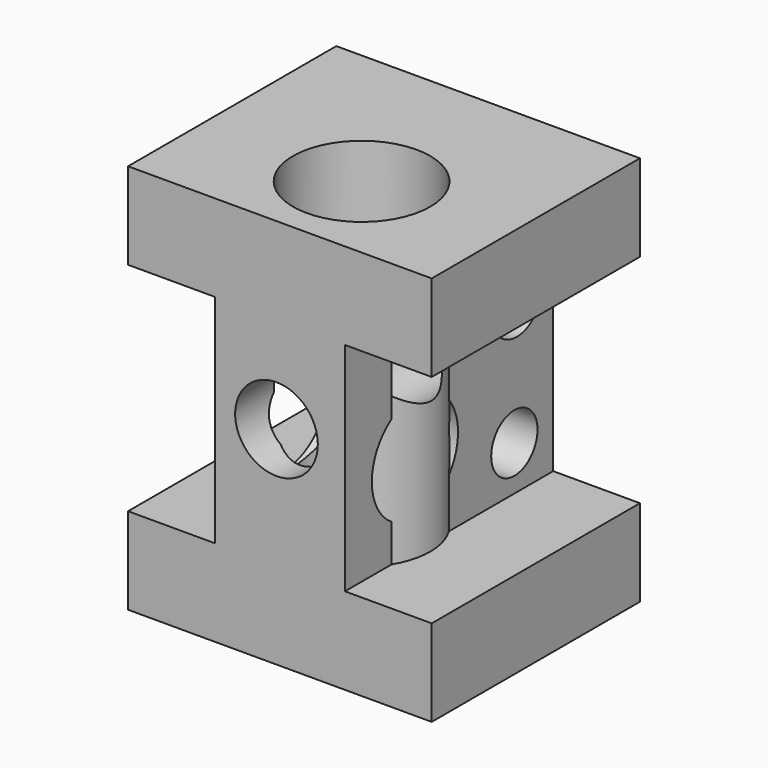
from build123d import *

# Parameters (mm, degrees)
F1_DEPTH  = 76.2
F2_R      = 15.7651741011
F3_DEPTH  = 63.501
F4_R      = 8.4797951308
F5_DEPTH  = 101.6
F6_R      = 9.0350925168
F7_DEPTH  = 101.6
F8_R      = 20.0966773981
F9_DEPTH  = 254
F10_R     = 12.1029149544
F11_DEPTH = 152.4


# Not quite as in the source:
# - a feature names something its author has since deleted; it is built from what else it names


with BuildPart() as f1:
    # F0 (on Front) → F1 (new body)
    with BuildSketch(Plane.XZ):
        Polygon((-39.3429771781, -29.9157751362), (-39.3429771781, -55.3157751362), (49.5570228219, -55.3157751362), (49.5570228219, -29.9157751362), (24.1570228219, -29.9157751362), (24.1570228219, 33.5842248638), (49.5570228219, 33.5842248638), (49.5570228219, 58.9842248638), (-39.3429771781, 58.9842248638), (-39.3429771781, 33.5842248638), (-13.9429771781, 33.5842248638), (-13.9429771781, -29.9157751362), align=None)
    extrude(amount=F1_DEPTH)

    # F2 (on face) → F3 (cut, through all)
    with BuildSketch(Plane.YZ.offset(24.1570228219)):
        with Locations((-50.584128027, -5.7007628794)):
            Circle(F2_R)
    extrude(amount=-F3_DEPTH, mode=Mode.SUBTRACT)

    # F4 (on face) → F5 (cut)
    with BuildSketch(Plane(origin=(-13.9429771781, 0, 0), x_dir=(0, -1, 0), z_dir=(-1, 0, 0))):
        with Locations((14.2035768056, -16.88193849)):
            Circle(F4_R)
    extrude(amount=-F5_DEPTH, mode=Mode.SUBTRACT)

    # F6 (on face) → F7 (cut)
    with BuildSketch(Plane(origin=(-13.9429771781, 0, 0), x_dir=(0, -1, 0), z_dir=(-1, 0, 0))):
        with Locations((13.3194467053, 19.1170163453)):
            Circle(F6_R)
    extrude(amount=-F7_DEPTH, mode=Mode.SUBTRACT)

    # F8 (on face) → F9 (cut)
    with BuildSketch(Plane(origin=(0, 0, -55.3157751362), x_dir=(1, 0, 0), z_dir=(0, 0, -1))):
        with Locations((7.0190951228, 48.6826710403)):
            Circle(F8_R)
    extrude(amount=-F9_DEPTH, mode=Mode.SUBTRACT)

    # F10 (on face) → F11 (cut)
    with BuildSketch(Plane.XZ.offset(76.2)):
        with Locations((4.1101346724, 5.3650285117)):
            Circle(F10_R)
    extrude(amount=-F11_DEPTH, mode=Mode.SUBTRACT)


solid = f1.part
